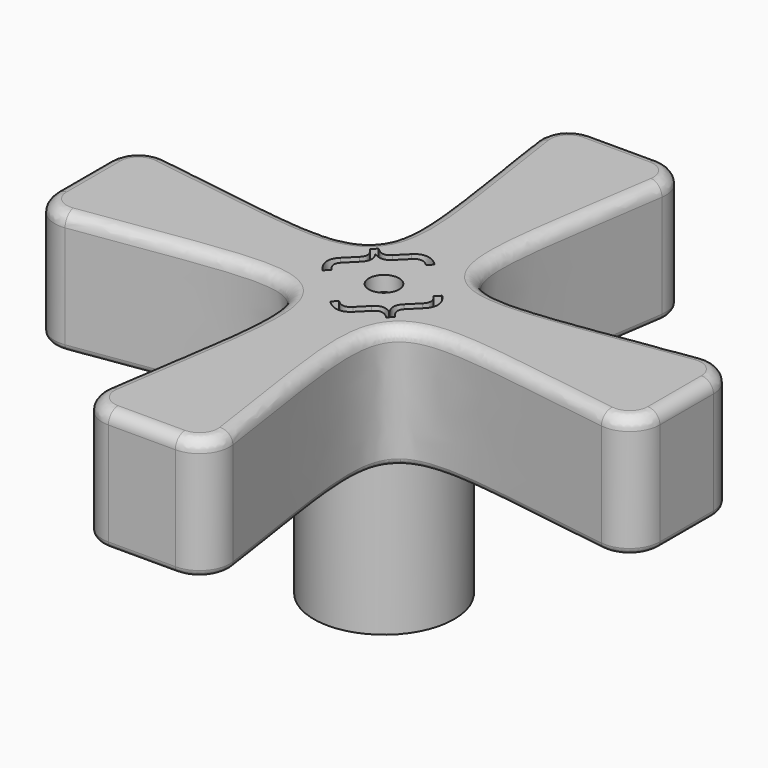
from build123d import *

# Parameters (mm, degrees)
F1_DEPTH     = 12.7
F2_R         = 7.366
F3_DEPTH     = 15.875
F4_R         = 1.5875
F4_TEXT_SIZE = 10.5833333333
F5_DEPTH     = 1.5875
F6_R         = 3.175
F7_R         = 1.27
F8_R         = 0.635
F9_R         = 1.5875
F10_DEPTH    = 19.05


# Not quite as in the source:
# - Text() gives the source's letters only with a copy of the font that has no kerning and outlines rounded to 1/6400 em; it was checked with that copy


with BuildPart() as f1:
    # F0 (on Top) → F1 (new body)
    with BuildSketch(Plane.XY):
        with BuildLine():
            add(Edge.make_bspline(
                [(-31.75, 7.14375), (-15.875, 5.08), (-0.7478201513, 0.7478201513), (-5.08, 15.875), (-7.14375, 31.75)],
                knots=[0, 0, 0, 0, 0.5, 1, 1, 1, 1], degree=3))
            Line((-31.75, 7.14375), (-31.75, -7.14375))
            add(Edge.make_bspline(
                [(-31.75, -7.14375), (-15.875, -5.08), (-0.7478201513, -0.7478201513), (-5.08, -15.875), (-7.14375, -31.75)],
                knots=[0, 0, 0, 0, 0.5, 1, 1, 1, 1], degree=3))
            Line((-7.14375, -31.75), (7.14375, -31.75))
            add(Edge.make_bspline(
                [(31.75, -7.14375), (15.875, -5.08), (0.7478201513, -0.7478201513), (5.08, -15.875), (7.14375, -31.75)],
                knots=[0, 0, 0, 0, 0.5, 1, 1, 1, 1], degree=3))
            Line((31.75, -7.14375), (31.75, 7.14375))
            add(Edge.make_bspline(
                [(31.75, 7.14375), (15.875, 5.08), (0.7478201513, 0.7478201513), (5.08, 15.875), (7.14375, 31.75)],
                knots=[0, 0, 0, 0, 0.5, 1, 1, 1, 1], degree=3))
            Line((7.14375, 31.75), (-7.14375, 31.75))
        make_face()
    extrude(amount=F1_DEPTH)

    # F2 (on face) → F3 (join)
    with BuildSketch(Plane(origin=(0, 0, 0), x_dir=(1, 0, 0), z_dir=(0, 0, -1))):
        Circle(F2_R)
    extrude(amount=F3_DEPTH)

    # F4 (on face) → F5 (cut)
    with BuildSketch(Plane.XY.offset(12.7)):
        Circle(F4_R)
        with Locations(Location((-6.8039998187, 2.4934768805), (0, 0, -45))):
            Text('{', F4_TEXT_SIZE, font='Open Sans', text_align=(TextAlign.LEFT, TextAlign.BOTTOM))
        with Locations(Location((-0.5677614691, -3.7427614691), (0, 0, -45))):
            Text('}', F4_TEXT_SIZE, font='Open Sans', text_align=(TextAlign.LEFT, TextAlign.BOTTOM))
    extrude(amount=-F5_DEPTH, mode=Mode.SUBTRACT)

    # F6
    f6_edges = [f1.edges().sort_by_distance(p)[0] for p in [
        (7.14375, -31.75, 6.35),
        (31.75, -7.14375, 6.35),
        (31.75, 7.14375, 6.35),
        (7.14375, 31.75, 6.35),
        (-7.14375, 31.75, 6.35),
        (-31.75, -7.14375, 6.35),
        (-31.75, 7.14375, 6.35),
        (-7.14375, -31.75, 6.35),
    ]]
    fillet(f6_edges, radius=F6_R)

    # F7
    f7_edges = [f1.edges().sort_by_distance(p)[0] for p in [
        (-5.61266, -5.61266, 12.7),
        (-5.61266, 5.61266, 12.7),
        (-30.658012, 5.906072, 12.7),
        (-5.906072, 30.658012, 12.7),
        (-31.75, 0, 12.7),
        (0, 31.75, 12.7),
        (-30.658012, -5.906072, 12.7),
        (5.906072, 30.658012, 12.7),
        (5.61266, 5.61266, 12.7),
        (-5.906072, -30.658012, 12.7),
        (30.658012, 5.906072, 12.7),
        (0, -31.75, 12.7),
        (31.75, 0, 12.7),
        (5.906072, -30.658012, 12.7),
        (30.658012, -5.906072, 12.7),
        (5.61266, -5.61266, 12.7),
    ]]
    fillet(f7_edges, radius=F7_R)

    # F8
    f8_edges = [f1.edges().sort_by_distance(p)[0] for p in [
        (-5.61266, 5.61266, 0),
        (-30.658012, 5.906072, 0),
        (-5.906072, 30.658012, 0),
        (-31.75, 0, 0),
        (0, 31.75, 0),
        (-30.658012, -5.906072, 0),
        (5.906072, 30.658012, 0),
        (-5.61266, -5.61266, 0),
        (5.61266, 5.61266, 0),
        (-5.906072, -30.658012, 0),
        (30.658012, 5.906072, 0),
        (0, -31.75, 0),
        (31.75, 0, 0),
        (5.906072, -30.658012, 0),
        (30.658012, -5.906072, 0),
        (5.61266, -5.61266, 0),
    ]]
    fillet(f8_edges, radius=F8_R)

    # F9 (on face) → F10 (cut)
    with BuildSketch(Plane(origin=(0, 0, -15.875), x_dir=(1, 0, 0), z_dir=(0, 0, -1))):
        Circle(F9_R)
    extrude(amount=-F10_DEPTH, mode=Mode.SUBTRACT)


solid = f1.part
